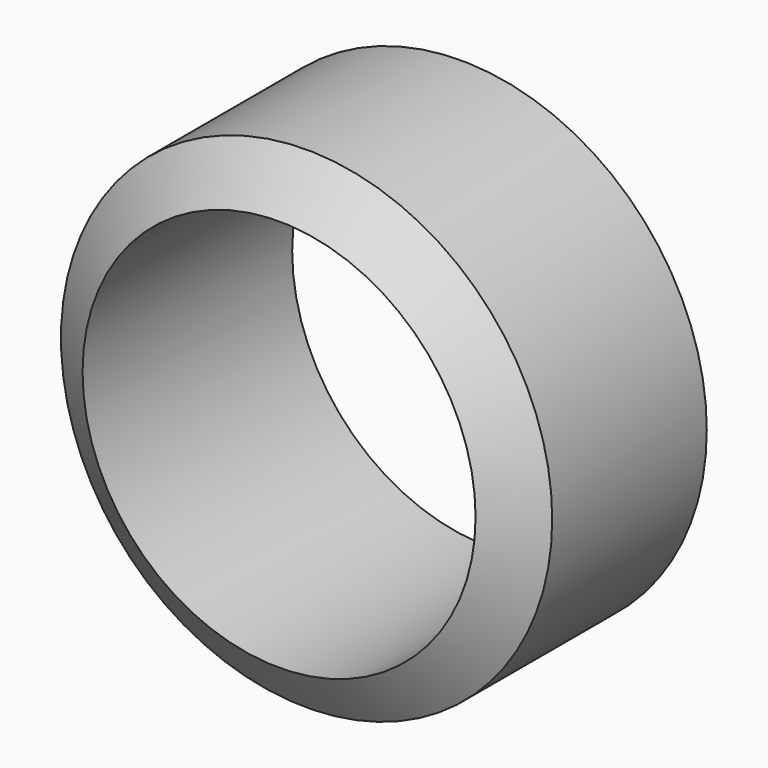
from build123d import *

# Parameters (mm, degrees)
F0_R       = 9.525
F0_R_2     = 7.62
F1_DEPTH   = 10.16
F2_SIZE2   = 1.333885
F2_SIZE    = 1.90499
F2_2_SIZE2 = 1.333885
F2_2_SIZE  = 1.90499


# Not quite as in the source:
# - a fillet or chamfer is up to 0.001 mm smaller than in the source, because OpenCascade refuses the exact size


with BuildPart() as f1:
    # F0 (on Front) → F1 (new body)
    with BuildSketch(Plane.XZ):
        Circle(F0_R)
        Circle(F0_R_2, mode=Mode.SUBTRACT)
    extrude(amount=F1_DEPTH)

    # F2 (size 1.905 and 1.3338953603 in the source; OpenCascade refuses exactly that, so slightly less here)
    f2_edges = [f1.edges().sort_by_distance(p)[0] for p in [
        (-9.525, -10.16, 0),
    ]]
    f2_side = f1.faces().sort_by_distance((-9.255592, -10.16, 0))[0]
    chamfer(f2_edges, length=F2_SIZE, length2=F2_SIZE2, reference=f2_side)

    # F2#2 (size 1.905 and 1.3338953603 in the source; OpenCascade refuses exactly that, so slightly less here)
    f2_2_edges = [f1.edges().sort_by_distance(p)[0] for p in [
        (-9.525, 0, 0),
    ]]
    f2_2_side = f1.faces().sort_by_distance((-9.255592, 0, 0))[0]
    chamfer(f2_2_edges, length=F2_2_SIZE, length2=F2_2_SIZE2, reference=f2_2_side)


solid = f1.part
